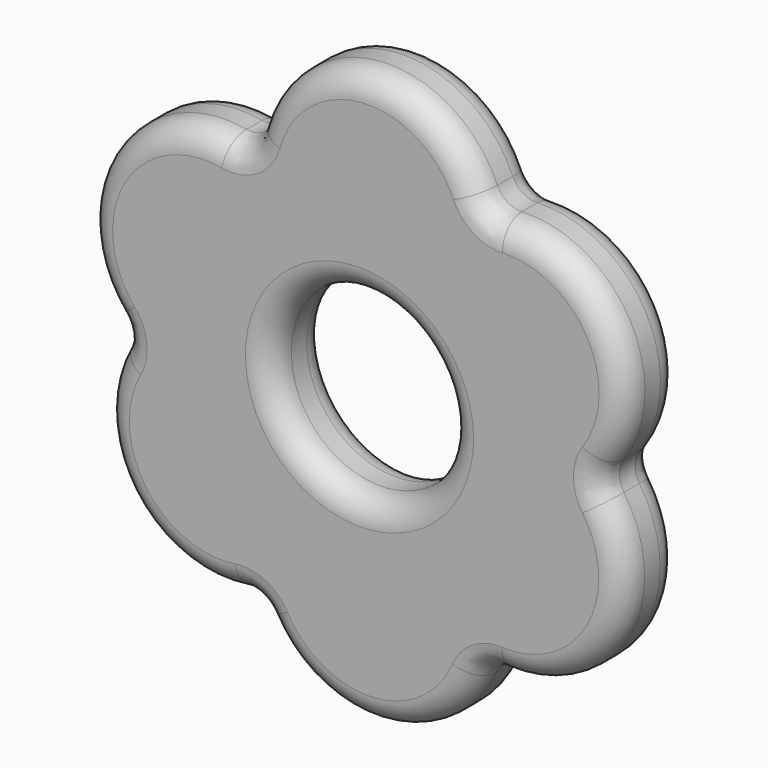
from build123d import *

# Parameters (mm, degrees)
F0_R     = 17.6390727143
F1_DEPTH = 14
F2_F1_R  = 5.08
F2_F2_R  = 5.08
F3_R     = 5.08


with BuildPart() as f1:
    # F0 (on Front) → F1 (new body)
    with BuildSketch(Plane.XZ):
        with BuildLine():
            ThreePointArc((-37.9055047614, 24.5986585343), (-67.052167974, 15.3393603296), (-62.285180516, -14.8688903687))
            ThreePointArc((-62.285180516, -14.8688903687), (-63.0184039924, -42.6940411891), (-36.6597824596, -51.6382966493))
            ThreePointArc((-36.6597824596, -51.6382966493), (-13.4512655262, -67.0051888725), (8.1018346172, -49.3915433369))
            ThreePointArc((8.1018346172, -49.3915433369), (33.4323385282, -37.8528169574), (29.9165229353, -10.2409413318))
            ThreePointArc((29.9165229353, -10.2409413318), (33.5542499923, 17.3551376779), (8.2749530245, 29.0056217735))
            ThreePointArc((8.2749530245, 29.0056217735), (-16.7086821727, 46.6430975568), (-37.9055047614, 24.5986585343))
        make_face()
        with Locations((-16.3055990562, -10.1388725882)):
            Circle(F0_R, mode=Mode.SUBTRACT)
    extrude(amount=F1_DEPTH)

    # F2: fillet of radius 5.08 on 12 edges, made by hand

    # F2_f1
    f2_f1_edges = [f1.edges().sort_by_distance(p)[0] for p in [
        (8.1018346172, -7, -49.3915433369),
        (29.9165229353, -7, -10.2409413318),
        (8.2749530245, -7, 29.0056217735),
        (-37.9055047614, -7, 24.5986585343),
        (-62.285180516, -7, -14.8688903687),
        (-36.6597824596, -7, -51.6382966493),
    ]]
    fillet(f2_f1_edges, radius=F2_F1_R)

    # F2_f2
    f2_f2_edges = [f1.edges().sort_by_distance(p)[0] for p in [
        (33.4323385282, 0, -37.8528169574),
        (33.4323385282, -14, -37.8528169574),
        (-15.9879244349, 0, 46.700686854),
        (-15.9879244349, -14, 46.700686854),
        (-63.0184039924, 0, -42.6940411891),
        (-63.0184039924, -14, -42.6940411891),
        (-63.7329960226, -14, -15.0178302431),
        (-37.3006996107, -14, -52.9450399419),
        (-63.7329960226, 0, -15.0178302431),
        (-37.3006996107, 0, -52.9450399419),
        (9.0489510326, -14, 30.2382125047),
        (-39.2545656407, -14, 26.7682533874),
        (9.0489510326, 0, 30.2382125047),
        (-39.2545656407, 0, 26.7682533874),
        (8.8703814336, -14, -50.6275403508),
        (31.3719756132, -14, -10.2441552956),
        (8.8703814336, 0, -50.6275403508),
        (31.3719756132, 0, -10.2441552956),
    ]]
    fillet(f2_f2_edges, radius=F2_F2_R)

    # F3
    f3_edges = [f1.edges().sort_by_distance(p)[0] for p in [
        (-33.944672, -14, -10.138873),
        (-33.944672, 0, -10.138873),
    ]]
    fillet(f3_edges, radius=F3_R)


solid = f1.part
